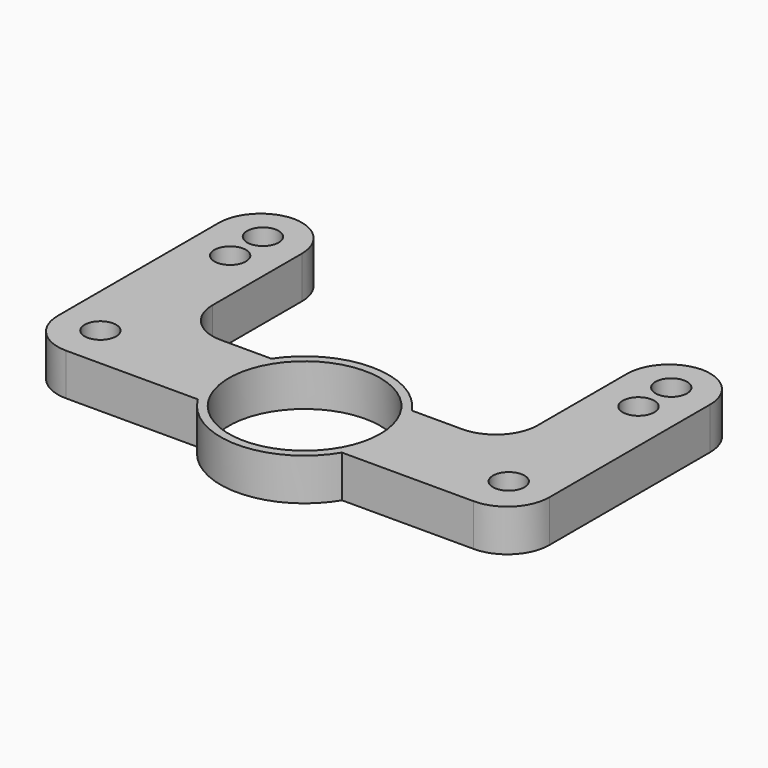
from build123d import *

# Parameters (mm, degrees)
F0_W        = 3.9569679648
F0_H        = 9.3060303107
F0_R        = 0.75
F1_DEPTH    = 2
F2_R        = 3.6
F3_DEPTH    = 25
F4_T1_DEPTH = 2
F4_T3_DEPTH = 12


# Not quite as in the source:
# - a fillet or chamfer that OpenCascade refuses, or shapes differently, is made with other operations: its cross-section is extruded or revolved along the edge and cut away or added


with BuildPart() as f1:
    # F0 (on Top) → F1 (new body)
    with BuildSketch(Plane.XY):
        with Locations((-9.7150150687, 6.8534435891)):
            Rectangle(F0_W, F0_H)
        with Locations((-9.7150150687, 7.7160103247)):
            Circle(F0_R, mode=Mode.SUBTRACT)
        with Locations((-9.7150150687, 9.6662240103)):
            Circle(F0_R, mode=Mode.SUBTRACT)
        with BuildLine():
            ThreePointArc((-3.4285871837, -2.0602887962), (-3.9991430252, 0.0827953119), (-3.3403764321, 2.2004284337))
            Line((-3.3403764321, 2.2004284337), (-7.7365310863, 2.2004284337))
            Line((-7.7365310863, 2.2004284337), (-11.693499051, 2.2004284337))
            Line((-11.693499051, 2.2004284337), (-11.693499051, -2.0602887962))
            Line((-11.693499051, -2.0602887962), (-3.4285871837, -2.0602887962))
        make_face()
        with Locations((-9.7150150687, 0)):
            Circle(F0_R, mode=Mode.SUBTRACT)
        with BuildLine():
            Line((3.3403764321, -2.0602887962), (3.3403764321, 2.2004284337))
            ThreePointArc((3.3403764321, 2.2004284337), (0, 4), (-3.3403764321, 2.2004284337))
            Line((-3.3403764321, 2.2004284337), (-3.3403764321, -2.0602887962))
            Line((-3.3403764321, -2.0602887962), (-3.4285871837, -2.0602887962))
            ThreePointArc((-3.4285871837, -2.0602887962), (0, -4), (3.4285871837, -2.0602887962))
            Line((3.4285871837, -2.0602887962), (3.3403764321, -2.0602887962))
        make_face()
        with BuildLine():
            ThreePointArc((3.3403764321, 2.2004284337), (3.8315470588, 1.1485848405), (4, 0))
            ThreePointArc((4, 0), (3.8545005341, -1.06903023), (3.4285871837, -2.0602887962))
            Line((3.4285871837, -2.0602887962), (11.693499051, -2.0602887962))
            Line((11.693499051, -2.0602887962), (11.693499051, 2.2004284337))
            Line((11.693499051, 2.2004284337), (7.7365310863, 2.2004284337))
            Line((7.7365310863, 2.2004284337), (3.3403764321, 2.2004284337))
        make_face()
        with Locations((9.7150150687, 0)):
            Circle(F0_R, mode=Mode.SUBTRACT)
        with Locations((9.7150150687, 6.8534435891)):
            Rectangle(F0_W, F0_H)
        with Locations((9.7150150687, 7.7160103247)):
            Circle(F0_R, mode=Mode.SUBTRACT)
        with Locations((9.7150150687, 9.6662240103)):
            Circle(F0_R, mode=Mode.SUBTRACT)
        with BuildLine():
            Line((-3.3403764321, -2.0602887962), (-3.3403764321, 2.2004284337))
            ThreePointArc((-3.3403764321, 2.2004284337), (-3.9991430252, 0.0827953119), (-3.4285871837, -2.0602887962))
            Line((-3.4285871837, -2.0602887962), (-3.3403764321, -2.0602887962))
        make_face()
        with BuildLine():
            ThreePointArc((3.4285871837, -2.0602887962), (3.8545005341, -1.06903023), (4, 0))
            ThreePointArc((4, 0), (3.8315470588, 1.1485848405), (3.3403764321, 2.2004284337))
            Line((3.3403764321, 2.2004284337), (3.3403764321, -2.0602887962))
            Line((3.3403764321, -2.0602887962), (3.4285871837, -2.0602887962))
        make_face()
    extrude(amount=F1_DEPTH)

    # F2 (on face) → F3 (cut)
    with BuildSketch(Plane.XY.offset(2)):
        Circle(F2_R)
    extrude(amount=-F3_DEPTH, mode=Mode.SUBTRACT)

    # F4: fillet of radius 2 on 8 edges, made by hand

    # F4_s2 → F4_t1 (join)
    with BuildSketch(Plane.XY):
        with BuildLine():
            ThreePointArc((-7.7365310863, 4.2004284337), (-7.1507446486, 2.7862148714), (-5.7365310863, 2.2004284337))
            Line((-5.7365310863, 2.2004284337), (-7.7365310863, 2.2004284337))
            Line((-7.7365310863, 2.2004284337), (-7.7365310863, 4.2004284337))
        make_face()
        with BuildLine():
            ThreePointArc((5.7365310863, 2.2004284337), (7.1507446486, 2.7862148714), (7.7365310863, 4.2004284337))
            Line((7.7365310863, 4.2004284337), (7.7365310863, 2.2004284337))
            Line((7.7365310863, 2.2004284337), (5.7365310863, 2.2004284337))
        make_face()
    extrude(amount=F4_T1_DEPTH)

    # F4_s4 → F4_t3 (cut)
    with BuildSketch(Plane.XY.offset(-5)):
        with BuildLine():
            ThreePointArc((9.693499051, 11.5064587444), (11.1077126134, 10.9206723068), (11.693499051, 9.5064587444))
            Line((11.693499051, 9.5064587444), (11.693499051, 11.5064587444))
            Line((11.693499051, 11.5064587444), (9.693499051, 11.5064587444))
        make_face()
        with BuildLine():
            ThreePointArc((7.7365310863, 9.5064587444), (8.3223175239, 10.9206723068), (9.7365310863, 11.5064587444))
            Line((9.7365310863, 11.5064587444), (7.7365310863, 11.5064587444))
            Line((7.7365310863, 11.5064587444), (7.7365310863, 9.5064587444))
        make_face()
        with BuildLine():
            ThreePointArc((-7.7365310863, 9.5064587444), (-8.3223175239, 10.9206723068), (-9.7365310863, 11.5064587444))
            Line((-9.7365310863, 11.5064587444), (-7.7365310863, 11.5064587444))
            Line((-7.7365310863, 11.5064587444), (-7.7365310863, 9.5064587444))
        make_face()
        with BuildLine():
            ThreePointArc((-9.693499051, 11.5064587444), (-11.1077126134, 10.9206723068), (-11.693499051, 9.5064587444))
            Line((-11.693499051, 9.5064587444), (-11.693499051, 11.5064587444))
            Line((-11.693499051, 11.5064587444), (-9.693499051, 11.5064587444))
        make_face()
        with BuildLine():
            ThreePointArc((-11.693499051, -0.0602887962), (-11.1077126134, -1.4745023586), (-9.693499051, -2.0602887962))
            Line((-9.693499051, -2.0602887962), (-11.693499051, -2.0602887962))
            Line((-11.693499051, -2.0602887962), (-11.693499051, -0.0602887962))
        make_face()
        with BuildLine():
            ThreePointArc((9.693499051, -2.0602887962), (11.1077126134, -1.4745023586), (11.693499051, -0.0602887962))
            Line((11.693499051, -0.0602887962), (11.693499051, -2.0602887962))
            Line((11.693499051, -2.0602887962), (9.693499051, -2.0602887962))
        make_face()
    extrude(amount=F4_T3_DEPTH, mode=Mode.SUBTRACT)


solid = f1.part
